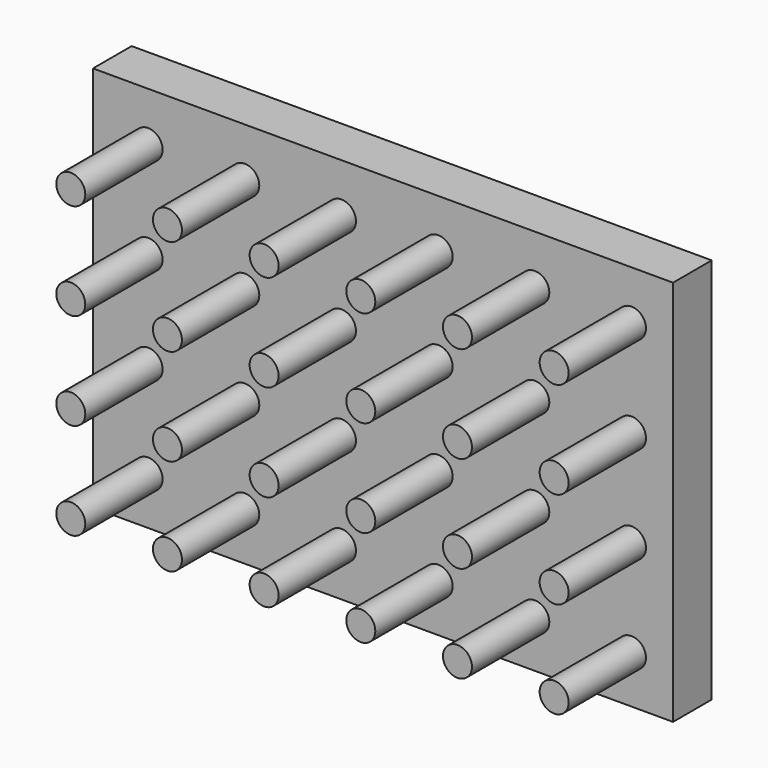
from build123d import *

# Parameters (mm, degrees)
F0_W     = 152.4
F0_H     = 101.6
F1_DEPTH = 12.7
F2_R     = 3.81
F3_DEPTH = 25.4


# Not quite as in the source:
# - a feature names something its author has since deleted; it is built from what else it names


with BuildPart() as f1:
    # F0 (on Front) → F1 (new body)
    with BuildSketch(Plane.XZ):
        with Locations((76.2, 50.8)):
            Rectangle(F0_W, F0_H)
    extrude(amount=F1_DEPTH)

    # F2 (on face) → F3 (join)
    with BuildSketch(Plane.XZ.offset(12.7)):
        with Locations((14.4803142175, 12.5110410154)):
            Circle(F2_R)
        with Locations((14.4803142175, 37.9110410154)):
            Circle(F2_R)
        with Locations((14.4803142175, 63.3110410154)):
            Circle(F2_R)
        with Locations((14.4803142175, 88.7110410154)):
            Circle(F2_R)
        with Locations((39.8803142175, 12.5110410154)):
            Circle(F2_R)
        with Locations((39.8803142175, 37.9110410154)):
            Circle(F2_R)
        with Locations((39.8803142175, 63.3110410154)):
            Circle(F2_R)
        with Locations((39.8803142175, 88.7110410154)):
            Circle(F2_R)
        with Locations((65.2803142175, 12.5110410154)):
            Circle(F2_R)
        with Locations((65.2803142175, 37.9110410154)):
            Circle(F2_R)
        with Locations((65.2803142175, 63.3110410154)):
            Circle(F2_R)
        with Locations((65.2803142175, 88.7110410154)):
            Circle(F2_R)
        with Locations((90.6803142175, 12.5110410154)):
            Circle(F2_R)
        with Locations((90.6803142175, 37.9110410154)):
            Circle(F2_R)
        with Locations((90.6803142175, 63.3110410154)):
            Circle(F2_R)
        with Locations((90.6803142175, 88.7110410154)):
            Circle(F2_R)
        with Locations((116.0803142175, 12.5110410154)):
            Circle(F2_R)
        with Locations((116.0803142175, 37.9110410154)):
            Circle(F2_R)
        with Locations((116.0803142175, 63.3110410154)):
            Circle(F2_R)
        with Locations((116.0803142175, 88.7110410154)):
            Circle(F2_R)
        with Locations((141.4803142175, 12.5110410154)):
            Circle(F2_R)
        with Locations((141.4803142175, 37.9110410154)):
            Circle(F2_R)
        with Locations((141.4803142175, 63.3110410154)):
            Circle(F2_R)
        with Locations((141.4803142175, 88.7110410154)):
            Circle(F2_R)
    extrude(amount=F3_DEPTH)


solid = f1.part
